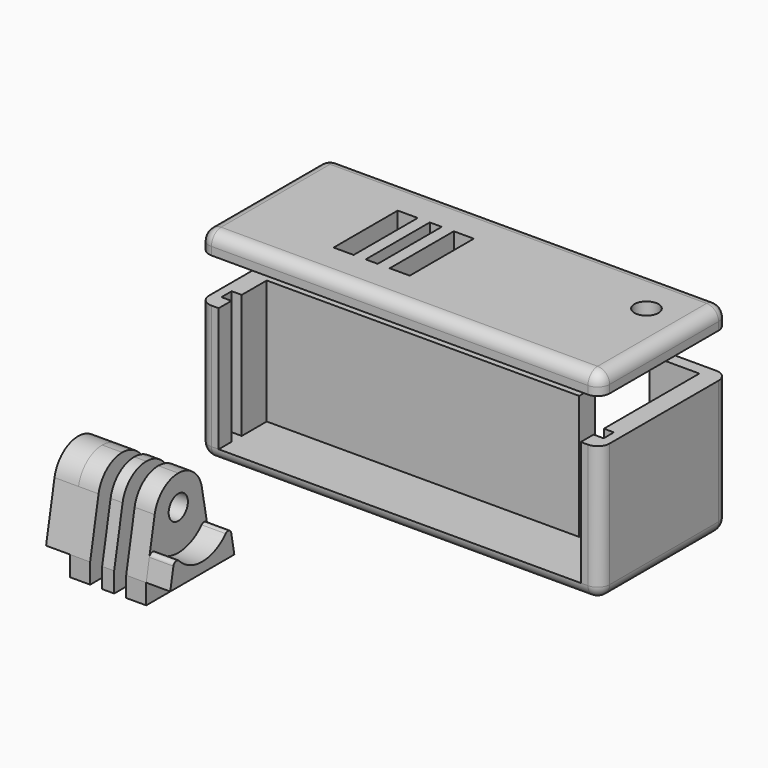
from build123d import *
from build123d import SkipClean  # not in build123d's __all__

# Parameters (mm, degrees)
F1_DEPTH     = 3
F2_DEPTH     = 34
F3_R         = 2.99999
F4_START     = 45
F4_DEPTH     = 5
F5_W         = 3
F5_H         = 20
F5_W_2       = 5
F5_R         = 3
F6_DEPTH     = 25
F7_R         = 3
F8_W         = 5
F8_H         = 20
F9_DEPTH     = 25
F8_W_2       = 3
F10_R        = 3
F11_DEPTH    = 25
F13_DEPTH    = 6
F14_T1_DEPTH = 11.6493534925
F15_R        = 3
F16_DEPTH    = 6
F18_DEPTH    = 4


# Not quite as in the source:
# - a fillet or chamfer that OpenCascade refuses, or shapes differently, is made with other operations: its cross-section is extruded or revolved along the edge and cut away or added
# - a fillet or chamfer is up to 0.001 mm smaller than in the source, because OpenCascade refuses the exact size
# - after a boolean that leaves OpenCascade's solid faulty, fix() repairs it


with BuildPart() as f1:
    # F0 (on Top) → F1 (new body)
    with BuildSketch(Plane.XY):
        Polygon((0, 40), (0, 0), (4.8, 0), (4.8, 4), (2.3, 4), (2.3, 7.2), (4.8, 7.2), (4.8, 15), (82.8, 15), (82.8, 20), (4.8, 20), (4.8, 37), (4.8, 40), align=None)
        Polygon((95.2, 4), (95.2, 0), (100, 0), (100, 40), (82.8, 40), (82.8, 37), (95.2, 37), (95.2, 7.2), (97.7, 7.2), (97.7, 4), align=None)
        Polygon((4.8, 4), (4.8, 0), (95.2, 0), (95.2, 4), (97.7, 4), (97.7, 7.2), (95.2, 7.2), (95.2, 37), (82.8, 37), (82.8, 40), (4.8, 40), (4.8, 37), (4.8, 20), (82.8, 20), (82.8, 15), (4.8, 15), (4.8, 7.2), (2.3, 7.2), (2.3, 4), align=None)
    extrude(amount=F1_DEPTH)

    # F0 (on Top) → F2 (join)
    with BuildSketch(Plane.XY):
        Polygon((0, 40), (0, 0), (4.8, 0), (4.8, 4), (2.3, 4), (2.3, 7.2), (4.8, 7.2), (4.8, 15), (82.8, 15), (82.8, 20), (4.8, 20), (4.8, 37), (4.8, 40), align=None)
        Polygon((95.2, 4), (95.2, 0), (100, 0), (100, 40), (82.8, 40), (82.8, 37), (95.2, 37), (95.2, 7.2), (97.7, 7.2), (97.7, 4), align=None)
    extrude(amount=F2_DEPTH)

    # F3 (radius 3 in the source; OpenCascade refuses exactly that, so slightly less here)
    f3_edges = [f1.edges().sort_by_distance(p)[0] for p in [
        (100, 20, 0),
        (50, 0, 0),
        (100, 0, 17),
        (0, 20, 0),
        (0, 0, 17),
        (0, 40, 17),
        (100, 40, 17),
        (50, 40, 0),
    ]]
    fillet(f3_edges, radius=F3_R)


with BuildPart() as f4:
    # F0 (on Top) → F4 (new body)
    with BuildSketch(Plane.XY.offset(F4_START)):
        Polygon((4.8, 4), (4.8, 0), (95.2, 0), (95.2, 4), (97.7, 4), (97.7, 7.2), (95.2, 7.2), (95.2, 37), (82.8, 37), (82.8, 40), (4.8, 40), (4.8, 37), (4.8, 20), (82.8, 20), (82.8, 15), (4.8, 15), (4.8, 7.2), (2.3, 7.2), (2.3, 4), align=None)
        Polygon((0, 40), (0, 0), (4.8, 0), (4.8, 4), (2.3, 4), (2.3, 7.2), (4.8, 7.2), (4.8, 15), (82.8, 15), (82.8, 20), (4.8, 20), (4.8, 37), (4.8, 40), align=None)
        Polygon((95.2, 4), (95.2, 0), (100, 0), (100, 40), (82.8, 40), (82.8, 37), (95.2, 37), (95.2, 7.2), (97.7, 7.2), (97.7, 4), align=None)
    extrude(amount=F4_DEPTH)

    # F5 (on face) → F6 (cut)
    with BuildSketch(Plane.XY.offset(50)):
        with Locations((35, 20)):
            Rectangle(F5_W, F5_H)
        with Locations((28, 20)):
            Rectangle(F5_W_2, F5_H)
        with Locations((42, 20)):
            Rectangle(F5_W_2, F5_H)
        with Locations((89.2, 28)):
            Circle(F5_R)
    extrude(amount=-F6_DEPTH, mode=Mode.SUBTRACT)

    # F7
    f7_edges = [f4.edges().sort_by_distance(p)[0] for p in [
        (0, 0, 47.5),
        (0, 40, 47.5),
        (100, 0, 47.5),
        (100, 40, 47.5),
        (50, 0, 50),
        (0, 20, 50),
        (50, 40, 50),
        (100, 20, 50),
    ]]
    fillet(f7_edges, radius=F7_R)


with BuildPart() as f9:
    # F8 (on Top) → F9 (new body)
    with BuildSketch(Plane.XY):
        with Locations((14.8477478921, -45.7968057692)):
            Rectangle(F8_W, F8_H)
    extrude(amount=F9_DEPTH)


with BuildPart() as f9b:
    # F8 (on Top) → F9, piece 2 (new body)
    with BuildSketch(Plane.XY):
        with Locations((28.8477478921, -45.7968057692)):
            Rectangle(F8_W, F8_H)
    extrude(amount=F9_DEPTH)


with BuildPart() as f9c:
    # F8 (on Top) → F9, piece 3 (new body)
    with BuildSketch(Plane.XY):
        with Locations((21.8477478921, -45.7968057692)):
            Rectangle(F8_W_2, F8_H)
    extrude(amount=F9_DEPTH)


with BuildPart() as f11_tool:
    # F10 (on face) → F11 (new body)
    with BuildSketch(Plane.YZ.offset(31.3477478921)):
        with BuildLine():
            Line((-55.7968057692, 5), (-53.1658797779, 18.8952592069))
            ThreePointArc((-53.1658797779, 18.8952592069), (-50.5814455648, 23.2755711428), (-45.7968057692, 25))
            Line((-45.7968057692, 25), (-55.7968057692, 25))
            Line((-55.7968057692, 25), (-55.7968057692, 5))
        make_face()
        with BuildLine():
            ThreePointArc((-45.7968057692, 25), (-41.0121659736, 23.2755711428), (-38.4277317605, 18.8952592069))
            Line((-38.4277317605, 18.8952592069), (-35.7968057692, 5))
            Line((-35.7968057692, 5), (-35.7968057692, 25))
            Line((-35.7968057692, 25), (-45.7968057692, 25))
        make_face()
        with Locations((-45.7968057692, 17.5)):
            Circle(F10_R)
    extrude(amount=-F11_DEPTH)


with BuildPart() as f9_1:
    add(f9.part, clean=False)

    # F11: cut by f11_tool
    add(f11_tool.part, mode=Mode.SUBTRACT)

    # F15 (on face) → F16 (join)
    with BuildSketch(Plane(origin=(12.3477478921, 0, 0), x_dir=(0, -1, 0), z_dir=(-1, 0, 0))):
        with BuildLine():
            Line((38.4277317605, 18.8952592069), (35.7968057692, 5))
            Line((35.7968057692, 5), (55.7968057692, 5))
            Line((55.7968057692, 5), (53.1658797779, 18.8952592069))
            ThreePointArc((53.1658797779, 18.8952592069), (45.7968057692, 25), (38.4277317605, 18.8952592069))
        make_face()
        with Locations((45.7968057692, 17.5)):
            Circle(F15_R, mode=Mode.SUBTRACT)
    with SkipClean():  # cleaning this boolean's faces spoils the solid; the shape is the same uncleaned
        extrude(amount=F16_DEPTH)

    # F17 (on face) → F18 (cut)
    with BuildSketch(Plane(origin=(6.3477478921, 0, 0), x_dir=(0, -1, 0), z_dir=(-1, 0, 0))):
        Polygon((49.8968057692, 19.8671361037), (45.7968057692, 22.2342722074), (41.6968057692, 19.8671361037), (41.6968057692, 15.1328638963), (45.7968057692, 12.7657277926), (49.8968057692, 15.1328638963), align=None)
    extrude(amount=-F18_DEPTH, mode=Mode.SUBTRACT)

    add(f9_1.part.fix(), mode=Mode.REPLACE)


with BuildPart() as f9b_1:
    add(f9b.part, clean=False)

    # F11: cut by f11_tool
    add(f11_tool.part, mode=Mode.SUBTRACT)

    # F12 (on face) → F13 (join)
    with BuildSketch(Plane.YZ.offset(31.3477478921)):
        with BuildLine():
            Line((-54.3963827366, 12.3963468003), (-55.7968057692, 5))
            Line((-55.7968057692, 5), (-35.7968057692, 5))
            Line((-35.7968057692, 5), (-37.1972288018, 12.3963468003))
            ThreePointArc((-37.1972288018, 12.3963468003), (-45.7968057692, 7.5), (-54.3963827366, 12.3963468003))
        make_face()
    extrude(amount=F13_DEPTH)

    # F14: fillet of radius 1 on 2 edges, made by hand

    # F14_s2 → F14_t1 (cut)
    with BuildSketch(Plane.YZ.offset(31.3477478921)):
        with BuildLine():
            ThreePointArc((-54.8167727352, 10.1760532544), (-54.1126804314, 10.9504691595), (-53.1035546463, 10.6727442668))
            ThreePointArc((-53.1035546463, 10.6727442668), (-53.7965246325, 11.4996251693), (-54.3963827366, 12.3963468003))
            Line((-54.3963827366, 12.3963468003), (-54.8167727352, 10.1760532544))
        make_face()
        with BuildLine():
            ThreePointArc((-36.7768388032, 10.1760532544), (-37.480931107, 10.9504691595), (-38.4900568921, 10.6727442668))
            ThreePointArc((-38.4900568921, 10.6727442668), (-37.797086906, 11.4996251693), (-37.1972288018, 12.3963468003))
            Line((-37.1972288018, 12.3963468003), (-36.7768388032, 10.1760532544))
        make_face()
    extrude(amount=F14_T1_DEPTH, mode=Mode.SUBTRACT)


with BuildPart() as f9c_1:
    add(f9c.part, clean=False)

    # F11: cut by f11_tool
    add(f11_tool.part, mode=Mode.SUBTRACT)


solid = Compound([f1.part, f4.part, f9_1.part, f9b_1.part, f9c_1.part])
